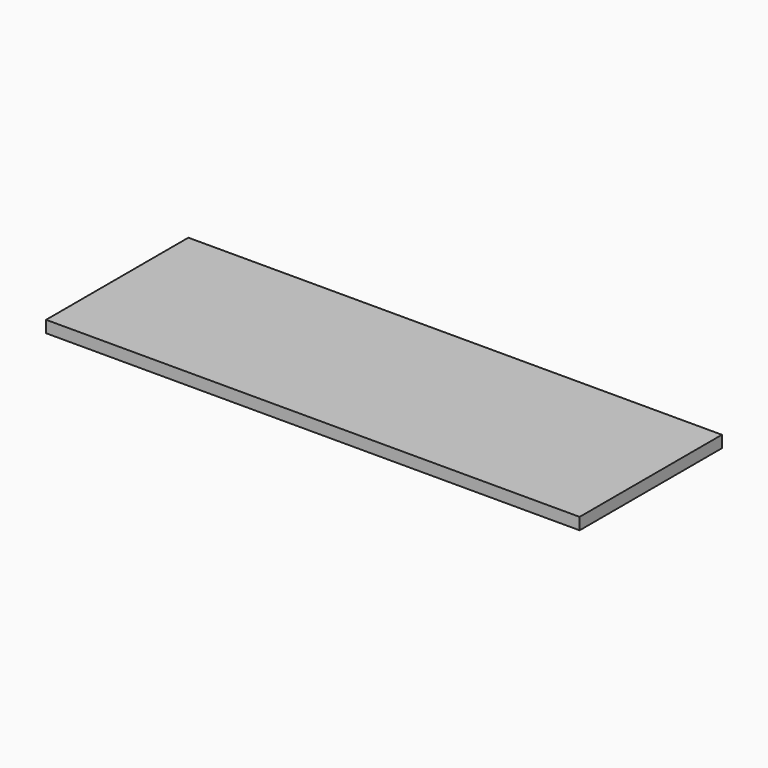
from build123d import *

# Parameters (mm, degrees)
F0_W     = 600
F0_H     = 40
F1_DEPTH = 1800


# Not quite as in the source:
# - a feature of the source that left no trace in its solid (it failed there, or was rolled back) is left out


with BuildPart() as f1:
    # F0 (on Right) → F1 (new body)
    with BuildSketch(Plane.YZ):
        with Locations((-300, 20)):
            Rectangle(F0_W, F0_H)
    extrude(amount=F1_DEPTH)


solid = f1.part
